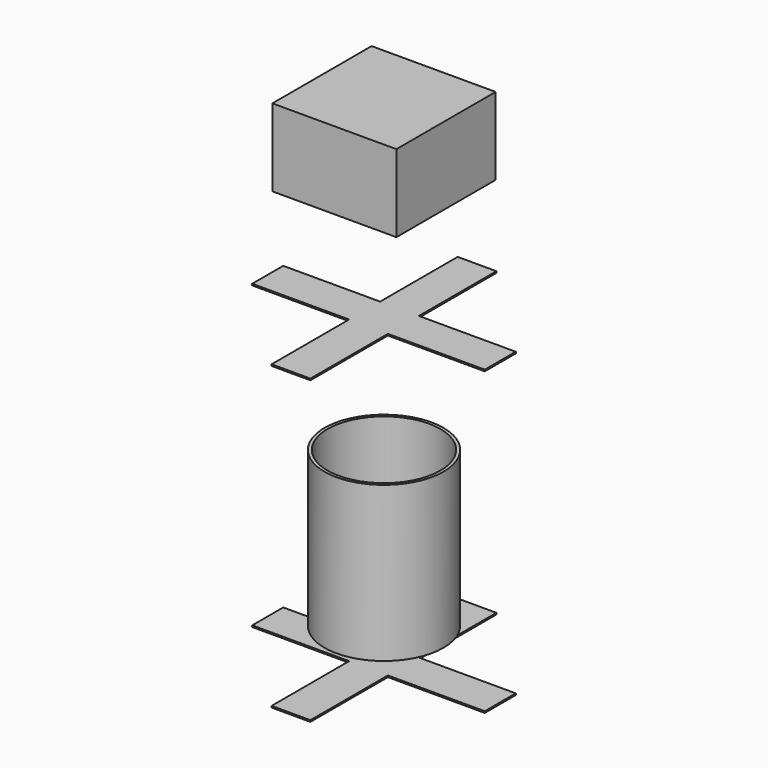
from build123d import *

# Parameters (mm, degrees)
F0_R      = 38.3718169686
F1_DEPTH  = 100
F2_R      = 36.3933090035
F3_DEPTH  = 100
F5_W      = 80
F5_H      = 80
F6_DEPTH  = 50
F11_W     = 62.5
F11_H     = 25
F11_W_2   = 25
F11_H_2   = 62.5
F12_DEPTH = 1
F14_W     = 62.5
F14_H     = 25
F14_W_2   = 25
F14_H_2   = 62.5
F15_DEPTH = 1


# Not quite as in the source:
# - the program builds the solid bodies; features that only make, move or delete a surface that nothing else refers to are left out


with BuildPart() as f1:
    # F0 (on Top) → F1 (new body)
    with BuildSketch(Plane.XY):
        Circle(F0_R)
    extrude(amount=-F1_DEPTH)

    # F2 (on face) → F3 (cut)
    with BuildSketch(Plane.XY):
        Circle(F2_R)
    extrude(amount=-F3_DEPTH, mode=Mode.SUBTRACT)


with BuildPart() as f6:
    # F5 (on offset) → F6 (new body)
    with BuildSketch(Plane.XY.offset(150)):
        Rectangle(F5_W, F5_H)
    extrude(amount=F6_DEPTH)


with BuildPart() as f12:
    # F11 (on offset) → F12 (new body)
    with BuildSketch(Plane.XY.offset(75)):
        with Locations((-43.75, 0)):
            Rectangle(F11_W, F11_H)
        with Locations((0, 43.75)):
            Rectangle(F11_W_2, F11_H_2)
        Rectangle(F11_W_2, F11_H)
        with Locations((43.75, 0)):
            Rectangle(F11_W, F11_H)
        with Locations((0, -43.75)):
            Rectangle(F11_W_2, F11_H_2)
    extrude(amount=-F12_DEPTH)


with BuildPart() as f15:
    # F14 (on offset) → F15 (new body)
    with BuildSketch(Plane.XY.offset(-120)):
        with Locations((43.75, 0)):
            Rectangle(F14_W, F14_H)
        Rectangle(F14_W_2, F14_H)
        with Locations((0, 43.75)):
            Rectangle(F14_W_2, F14_H_2)
        with Locations((-43.75, 0)):
            Rectangle(F14_W, F14_H)
        with Locations((0, -43.75)):
            Rectangle(F14_W_2, F14_H_2)
    extrude(amount=F15_DEPTH)


solid = Compound([f1.part, f6.part, f12.part, f15.part])
